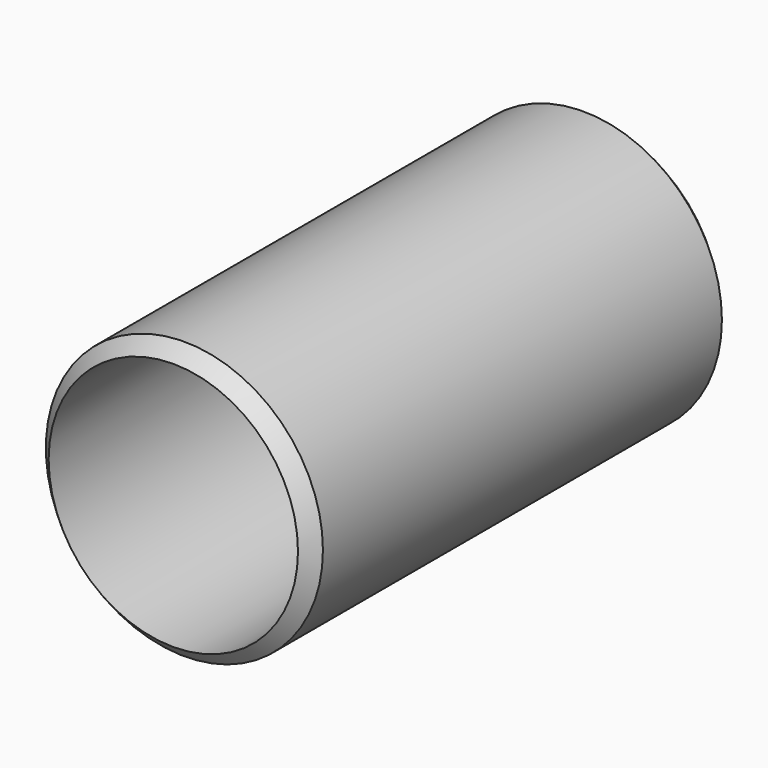
from build123d import *

# Parameters (mm, degrees)
F0_R     = 25.4
F0_R_2   = 23.495
F1_DEPTH = 50.8
F3_D     = 45.72


# Not quite as in the source:
# - a fillet or chamfer that OpenCascade refuses, or shapes differently, is made with other operations: its cross-section is extruded or revolved along the edge and cut away or added


with BuildPart() as f1:
    # F0 (on Front) → F1 (new body, symmetric)
    with BuildSketch(Plane.XZ):
        Circle(F0_R)
        Circle(F0_R_2, mode=Mode.SUBTRACT)
        Circle(F0_R_2)
    extrude(amount=F1_DEPTH, both=True)

    # F3 (through all)
    with Locations(Plane.XZ.offset(50.8)):
        with Locations((0, 0)):
            Hole(F3_D / 2)

    # F4: chamfer of 5.08 on 3 edges, made by hand

    # F4_s1 → F4_t2 (revolve, cut)
    with BuildSketch(Plane.XY):
        Polygon((25.4, 45.72), (20.32, 50.8), (25.4, 50.8), align=None)
    revolve(axis=Axis((0, 50.8, 0), (0, -1, 0)), mode=Mode.SUBTRACT)

    # F4_s3 → F4_t4 (revolve, cut)
    with BuildSketch(Plane.XY):
        Polygon((25.4, -45.72), (20.32, -50.8), (25.4, -50.8), align=None)
    revolve(axis=Axis((0, -50.8, 0), (0, -1, 0)), mode=Mode.SUBTRACT)


solid = f1.part
